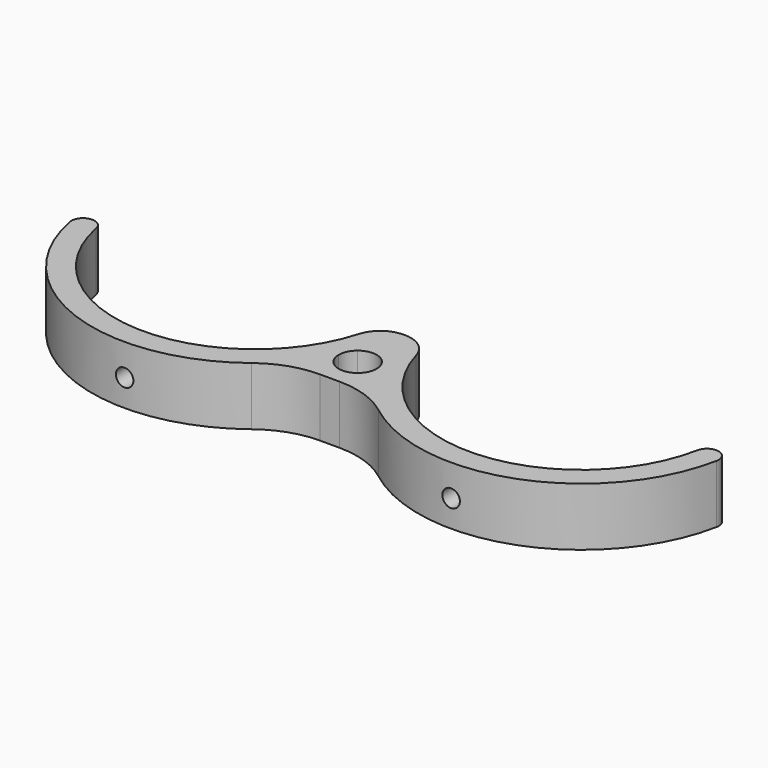
from build123d import *

# Parameters (mm, degrees)
F1_DEPTH = 10
F2_R     = 5
F3_R     = 15
F4_R     = 1.99999
F5_R     = 1.5
F6_DEPTH = 70
F7_DEPTH = 2


# Not quite as in the source:
# - a fillet or chamfer is up to 0.001 mm smaller than in the source, because OpenCascade refuses the exact size
# - a feature names something its author has since deleted; it is built from what else it names


with BuildPart() as f1:
    # F0 (on Top) → F1 (new body)
    with BuildSketch(Plane.XY):
        with BuildLine():
            ThreePointArc((-4.8029336206, -42.6810749437), (-6.0551509394, -44.3903306382), (-7.4330361988, -46))
            Line((-7.4330361988, -46), (-2.8867513459, -46))
            Line((-2.8867513459, -46), (-3.1754264805, -45.5))
            Line((-3.1754264805, -45.5), (-3.7929698378, -44.4303835293))
            Line((-3.7929698378, -44.4303835293), (-4.8029336206, -42.6810749437))
        make_face()
        with BuildLine():
            Line((4.1882382004, -30), (0.1611781858, -30))
            ThreePointArc((0.1611781858, -30), (0.4999682243, -32.2676609927), (1.0231580796, -34.5))
            Line((1.0231580796, -34.5), (3.1754264805, -34.5))
            Line((3.1754264805, -34.5), (6.3508529611, -40))
            Line((6.3508529611, -40), (4.8029336206, -42.6810749437))
            ThreePointArc((4.8029336206, -42.6810749437), (6.0551509394, -44.3903306382), (7.4330361988, -46))
            Line((7.4330361988, -46), (8, -46))
            Line((8, -46), (8, -40.2664991614))
            ThreePointArc((8, -40.2664991614), (5.5007140279, -35.3535699402), (4.1882382004, -30))
        make_face()
        with BuildLine():
            Line((-51.8117617996, -30), (-55.8388218142, -30))
            ThreePointArc((-55.8388218142, -30), (-36.7874899568, -53.585334684), (-7.4330361988, -46))
            Line((-7.4330361988, -46), (-8, -46))
            Line((-8, -46), (-8, -40.2664991614))
            ThreePointArc((-8, -40.2664991614), (-33.4756399865, -50.367014502), (-51.8117617996, -30))
        make_face()
        with BuildLine():
            ThreePointArc((51.8117617996, -30), (33.4756399865, -50.367014502), (8, -40.2664991614))
            Line((8, -40.2664991614), (8, -46))
            Line((8, -46), (7.4330361988, -46))
            ThreePointArc((7.4330361988, -46), (36.7874899568, -53.585334684), (55.8388218142, -30))
            Line((55.8388218142, -30), (51.8117617996, -30))
        make_face()
        with BuildLine():
            ThreePointArc((-4.1882382004, -30), (-5.5007140279, -35.3535699402), (-8, -40.2664991614))
            Line((-8, -40.2664991614), (-8, -46))
            Line((-8, -46), (-7.4330361988, -46))
            ThreePointArc((-7.4330361988, -46), (-6.0551509394, -44.3903306382), (-4.8029336206, -42.6810749437))
            Line((-4.8029336206, -42.6810749437), (-6.3508529611, -40))
            Line((-6.3508529611, -40), (-3.1754264805, -34.5))
            Line((-3.1754264805, -34.5), (-1.0231580796, -34.5))
            ThreePointArc((-1.0231580796, -34.5), (-0.4999682243, -32.2676609927), (-0.1611781858, -30))
            Line((-0.1611781858, -30), (-4.1882382004, -30))
        make_face()
        with BuildLine():
            Line((1.0231580796, -34.5), (-1.0231580796, -34.5))
            ThreePointArc((-1.0231580796, -34.5), (-1.4837475224, -35.993795336), (-2.0269826837, -37.4595588572))
            ThreePointArc((-2.0269826837, -37.4595588572), (0, -36.75), (2.0269826837, -37.4595588572))
            ThreePointArc((2.0269826837, -37.4595588572), (1.4837475224, -35.993795336), (1.0231580796, -34.5))
        make_face()
        with BuildLine():
            Line((2.8867513459, -46), (7.4330361988, -46))
            ThreePointArc((7.4330361988, -46), (6.0551509394, -44.3903306382), (4.8029336206, -42.6810749437))
            Line((4.8029336206, -42.6810749437), (3.917737902, -44.2142789029))
            Line((3.917737902, -44.2142789029), (3.1754264805, -45.5))
            Line((3.1754264805, -45.5), (2.8867513459, -46))
        make_face()
        with BuildLine():
            ThreePointArc((-2.0269826837, -37.4595588572), (-1.4837475224, -35.993795336), (-1.0231580796, -34.5))
            Line((-1.0231580796, -34.5), (-3.1754264805, -34.5))
            Line((-3.1754264805, -34.5), (-6.3508529611, -40))
            Line((-6.3508529611, -40), (-4.8029336206, -42.6810749437))
            ThreePointArc((-4.8029336206, -42.6810749437), (-3.9908775438, -41.4070135311), (-3.2487256059, -40.0910051512))
            ThreePointArc((-3.2487256059, -40.0910051512), (-2.9477791452, -38.631388254), (-2.0269826837, -37.4595588572))
        make_face()
        with BuildLine():
            Line((0.1611781858, -30), (-0.1611781858, -30))
            ThreePointArc((-0.1611781858, -30), (-0.4999682243, -32.2676609927), (-1.0231580796, -34.5))
            Line((-1.0231580796, -34.5), (1.0231580796, -34.5))
            ThreePointArc((1.0231580796, -34.5), (0.4999682243, -32.2676609927), (0.1611781858, -30))
        make_face()
        with BuildLine():
            Line((3.1754264805, -34.5), (1.0231580796, -34.5))
            ThreePointArc((1.0231580796, -34.5), (1.4837475224, -35.993795336), (2.0269826837, -37.4595588572))
            ThreePointArc((2.0269826837, -37.4595588572), (2.9283266315, -38.5902471355), (3.25, -40))
            ThreePointArc((3.25, -40), (3.2496813859, -40.0455070369), (3.2487256059, -40.0910051512))
            ThreePointArc((3.2487256059, -40.0910051512), (3.9908775438, -41.4070135311), (4.8029336206, -42.6810749437))
            Line((4.8029336206, -42.6810749437), (6.3508529611, -40))
            Line((6.3508529611, -40), (3.1754264805, -34.5))
        make_face()
        with BuildLine():
            ThreePointArc((-3.2487256059, -40.0910051512), (-3.9908775438, -41.4070135311), (-4.8029336206, -42.6810749437))
            Line((-4.8029336206, -42.6810749437), (-3.7929698378, -44.4303835293))
            Line((-3.7929698378, -44.4303835293), (-3.1754264805, -45.5))
            Line((-3.1754264805, -45.5), (3.1754264805, -45.5))
            Line((3.1754264805, -45.5), (3.917737902, -44.2142789029))
            Line((3.917737902, -44.2142789029), (4.8029336206, -42.6810749437))
            ThreePointArc((4.8029336206, -42.6810749437), (3.9908775438, -41.4070135311), (3.2487256059, -40.0910051512))
            ThreePointArc((3.2487256059, -40.0910051512), (0, -43.25), (-3.2487256059, -40.0910051512))
        make_face()
        Polygon((-3.1754264805, -45.5), (-2.8867513459, -46), (2.8867513459, -46), (3.1754264805, -45.5), align=None)
    extrude(amount=F1_DEPTH)

    # F2
    f2_edges = [f1.edges().sort_by_distance(p)[0] for p in [
        (-4.188238, -30, 5),
        (4.188238, -30, 5),
    ]]
    fillet(f2_edges, radius=F2_R)

    # F3
    f3_edges = [f1.edges().sort_by_distance(p)[0] for p in [
        (-7.433036, -46, 5),
        (7.433036, -46, 5),
    ]]
    fillet(f3_edges, radius=F3_R)

    # F4 (radius 2 in the source; OpenCascade refuses exactly that, so slightly less here)
    f4_edges = [f1.edges().sort_by_distance(p)[0] for p in [
        (-55.838822, -30, 5),
        (-51.811762, -30, 5),
        (51.811762, -30, 5),
        (55.838822, -30, 5),
    ]]
    fillet(f4_edges, radius=F4_R)

    # F5 (on Front) → F6 (cut)
    with BuildSketch(Plane.XZ):
        with Locations((-28, 4.6102153137)):
            Circle(F5_R)
        with Locations((28, 4.6102153137)):
            Circle(F5_R)
    extrude(amount=F6_DEPTH, mode=Mode.SUBTRACT)

    # F0 (on Top) → F7 (cut)
    with BuildSketch(Plane.XY):
        with BuildLine():
            Line((3.1754264805, -34.5), (1.0231580796, -34.5))
            ThreePointArc((1.0231580796, -34.5), (1.4837475224, -35.993795336), (2.0269826837, -37.4595588572))
            ThreePointArc((2.0269826837, -37.4595588572), (2.9283266315, -38.5902471355), (3.25, -40))
            ThreePointArc((3.25, -40), (3.2496813859, -40.0455070369), (3.2487256059, -40.0910051512))
            ThreePointArc((3.2487256059, -40.0910051512), (3.9908775438, -41.4070135311), (4.8029336206, -42.6810749437))
            Line((4.8029336206, -42.6810749437), (6.3508529611, -40))
            Line((6.3508529611, -40), (3.1754264805, -34.5))
        make_face()
        with BuildLine():
            Line((1.0231580796, -34.5), (-1.0231580796, -34.5))
            ThreePointArc((-1.0231580796, -34.5), (-1.4837475224, -35.993795336), (-2.0269826837, -37.4595588572))
            ThreePointArc((-2.0269826837, -37.4595588572), (0, -36.75), (2.0269826837, -37.4595588572))
            ThreePointArc((2.0269826837, -37.4595588572), (1.4837475224, -35.993795336), (1.0231580796, -34.5))
        make_face()
        with BuildLine():
            ThreePointArc((-2.0269826837, -37.4595588572), (-1.4837475224, -35.993795336), (-1.0231580796, -34.5))
            Line((-1.0231580796, -34.5), (-3.1754264805, -34.5))
            Line((-3.1754264805, -34.5), (-6.3508529611, -40))
            Line((-6.3508529611, -40), (-4.8029336206, -42.6810749437))
            ThreePointArc((-4.8029336206, -42.6810749437), (-3.9908775438, -41.4070135311), (-3.2487256059, -40.0910051512))
            ThreePointArc((-3.2487256059, -40.0910051512), (-2.9477791452, -38.631388254), (-2.0269826837, -37.4595588572))
        make_face()
        with BuildLine():
            ThreePointArc((-3.2487256059, -40.0910051512), (-3.9908775438, -41.4070135311), (-4.8029336206, -42.6810749437))
            Line((-4.8029336206, -42.6810749437), (-3.7929698378, -44.4303835293))
            Line((-3.7929698378, -44.4303835293), (-3.1754264805, -45.5))
            Line((-3.1754264805, -45.5), (3.1754264805, -45.5))
            Line((3.1754264805, -45.5), (3.917737902, -44.2142789029))
            Line((3.917737902, -44.2142789029), (4.8029336206, -42.6810749437))
            ThreePointArc((4.8029336206, -42.6810749437), (3.9908775438, -41.4070135311), (3.2487256059, -40.0910051512))
            ThreePointArc((3.2487256059, -40.0910051512), (0, -43.25), (-3.2487256059, -40.0910051512))
        make_face()
    extrude(amount=F7_DEPTH, mode=Mode.SUBTRACT)


solid = f1.part
